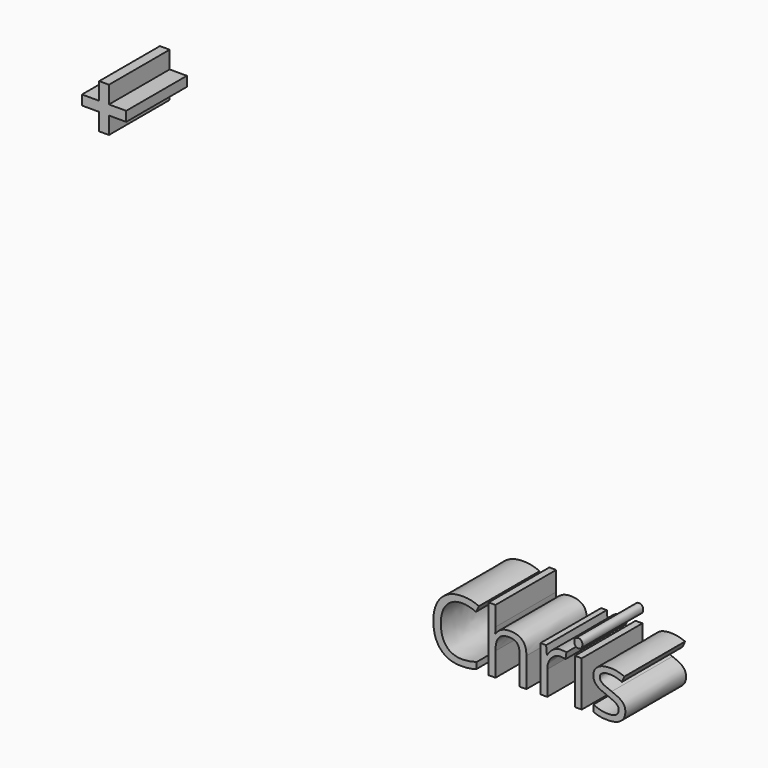
from build123d import *

# Parameters (mm, degrees)
F0_TEXT_SIZE = 14.1236109711
F1_DEPTH     = 12.7
F2_TEXT_SIZE = 15.269090525
F3_DEPTH     = 12.7


# Not quite as in the source:
# - Text() gives the source's letters only with a copy of the font that has no kerning and outlines rounded to 1/6400 em; it was checked with that copy


with BuildPart() as f1:
    # F0 (on Front) → F1 (new body)
    with BuildSketch(Plane.XZ):
        with Locations((-16.9615740506, 0)):
            Text('Chris', F0_TEXT_SIZE, font='Open Sans', text_align=(TextAlign.LEFT, TextAlign.BOTTOM))
    extrude(amount=F1_DEPTH)


with BuildPart() as f3:
    # F2 (on Front) → F3 (new body)
    with BuildSketch(Plane.XZ):
        with Locations((-75.5819678307, 57.2590641677)):
            Text('+', F2_TEXT_SIZE, font='Open Sans', font_style=FontStyle.BOLD, text_align=(TextAlign.LEFT, TextAlign.BOTTOM))
    extrude(amount=F3_DEPTH)


solid = Compound([f1.part, f3.part])
